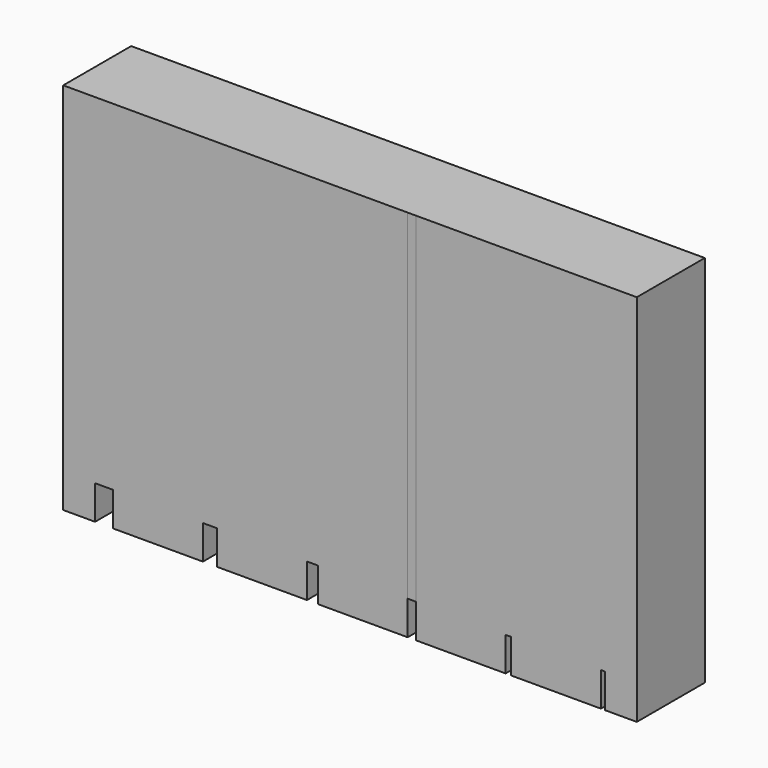
from build123d import *

# Parameters (mm, degrees)
F0_W     = 2.38125
F0_H     = 6.35
F0_W_2   = 1.3462
F0_W_3   = 6.71068
F0_W_4   = 1.0668
F0_W_5   = 0.8128
F0_W_6   = 0.4064
F0_W_7   = 0.3048
F1_DEPTH = 25.4
F2_DEPTH = 2.54


# Not quite as in the source:
# - ends of sketch curves that miss each other by under 0.0002 mm in the source are joined


with BuildPart() as f1:
    # F0 (on Top) → F1 (new body)
    with BuildSketch(Plane.XY):
        with Locations((-22.328797859, -3.175)):
            Rectangle(F0_W, F0_H)
        with Locations((18.152452141, -3.175)):
            Rectangle(F0_W, F0_H)
        with Locations((-20.465072859, -3.175)):
            Rectangle(F0_W_2, F0_H)
        with Locations((-16.436632859, -3.175)):
            Rectangle(F0_W_3, F0_H)
        with Locations((-12.547892859, -3.175)):
            Rectangle(F0_W_4, F0_H)
        with Locations((-8.659152859, -3.175)):
            Rectangle(F0_W_3, F0_H)
        with Locations((-4.897412859, -3.175)):
            Rectangle(F0_W_5, F0_H)
        with Locations((-1.135672859, -3.175)):
            Rectangle(F0_W_3, F0_H)
        Polygon((2.829267141, 0), (2.219667141, 0), (2.219667141, -6.3499879551), (2.829267141, -6.35), align=None)
        with Locations((6.184607141, -3.175)):
            Rectangle(F0_W_3, F0_H)
        with Locations((9.743147141, -3.175)):
            Rectangle(F0_W_6, F0_H)
        with Locations((13.301687141, -3.175)):
            Rectangle(F0_W_3, F0_H)
        with Locations((16.809427141, -3.175)):
            Rectangle(F0_W_7, F0_H)
    extrude(amount=F1_DEPTH)

    # F0 (on Top) → F2 (join)
    with BuildSketch(Plane.XY):
        with Locations((-22.328797859, -3.175)):
            Rectangle(F0_W, F0_H)
        with Locations((-16.436632859, -3.175)):
            Rectangle(F0_W_3, F0_H)
        with Locations((-8.659152859, -3.175)):
            Rectangle(F0_W_3, F0_H)
        with Locations((-1.135672859, -3.175)):
            Rectangle(F0_W_3, F0_H)
        with Locations((6.184607141, -3.175)):
            Rectangle(F0_W_3, F0_H)
        with Locations((13.301687141, -3.175)):
            Rectangle(F0_W_3, F0_H)
        with Locations((18.152452141, -3.175)):
            Rectangle(F0_W, F0_H)
    extrude(amount=-F2_DEPTH)


solid = f1.part
